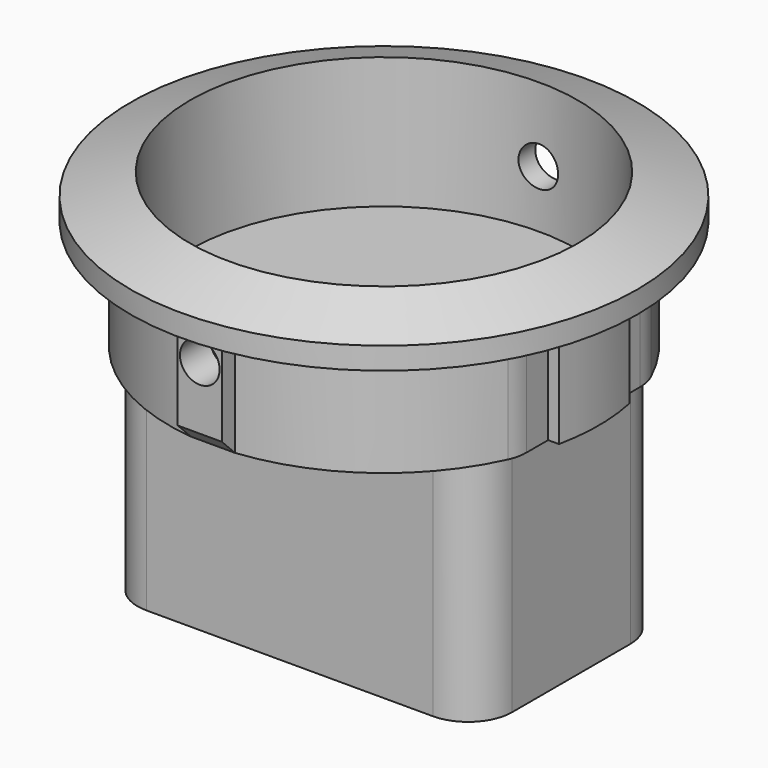
from build123d import *

# Parameters (mm, degrees)
F0_R      = 11.5
F1_DEPTH  = 2
F3_DEPTH  = 5
F5_DEPTH  = 10.5
F6_W      = 0.8
F6_H      = 5
F7_DEPTH  = 5
F8_R      = 8.8
F9_DEPTH  = 6
F11_R     = 2
F12_SIZE  = 0.75
F13_R     = 0.9
F14_DEPTH = 21.9495823706


# Not quite as in the source:
# - a fillet or chamfer that OpenCascade refuses, or shapes differently, is made with other operations: its cross-section is extruded or revolved along the edge and cut away or added


with BuildPart() as f1:
    # F0 (on Top) → F1 (new body)
    with BuildSketch(Plane.XY):
        Circle(F0_R)
    extrude(amount=F1_DEPTH)

    # F2 (on face) → F3 (join)
    with BuildSketch(Plane(origin=(0, 0, 0), x_dir=(1, 0, 0), z_dir=(0, 0, -1))):
        with BuildLine():
            Line((-9.05, -2), (-9.05, -3.6276714294))
            ThreePointArc((-9.05, -3.6276714294), (0, -9.75), (9.05, -3.6276714294))
            Line((9.05, -3.6276714294), (9.05, -2))
            Line((9.05, -2), (9.05, 2))
            Line((9.05, 2), (9.05, 3.6276714294))
            ThreePointArc((9.05, 3.6276714294), (5.8706571109, 7.7844643416), (1, 9.6985823706))
            Line((1, 9.6985823706), (1, 10.4485823706))
            Line((1, 10.4485823706), (-1, 10.4485823706))
            Line((-1, 10.4485823706), (-1, 9.6985823706))
            ThreePointArc((-1, 9.6985823706), (-5.8706571109, 7.7844643416), (-9.05, 3.6276714294))
            Line((-9.05, 3.6276714294), (-9.05, 2))
            Line((-9.05, 2), (-9.05, -2))
        make_face()
        with BuildLine():
            Line((-9.542667342, -2), (-9.05, -2))
            Line((-9.05, -2), (-9.05, 2))
            Line((-9.05, 2), (-9.542667342, 2))
            ThreePointArc((-9.542667342, 2), (-9.75, 0), (-9.542667342, -2))
        make_face()
        with BuildLine():
            Line((9.05, 2), (9.05, -2))
            Line((9.05, -2), (9.542667342, -2))
            ThreePointArc((9.542667342, -2), (9.75, 0), (9.542667342, 2))
            Line((9.542667342, 2), (9.05, 2))
        make_face()
    extrude(amount=F3_DEPTH)

    # F4 (on face) → F5 (join)
    with BuildSketch(Plane(origin=(0, 0, -5), x_dir=(1, 0, 0), z_dir=(0, 0, -1))):
        with BuildLine():
            Line((6.5, 5.35), (-6.5, 5.35))
            ThreePointArc((-6.5, 5.35), (-7.9142135624, 4.7642135624), (-8.5, 3.35))
            Line((-8.5, 3.35), (-8.5, -3.35))
            ThreePointArc((-8.5, -3.35), (-7.9142135624, -4.7642135624), (-6.5, -5.35))
            Line((-6.5, -5.35), (6.5, -5.35))
            ThreePointArc((6.5, -5.35), (7.9142135624, -4.7642135624), (8.5, -3.35))
            Line((8.5, -3.35), (8.5, 3.35))
            ThreePointArc((8.5, 3.35), (7.9142135624, 4.7642135624), (6.5, 5.35))
        make_face()
    extrude(amount=F5_DEPTH)

    # F6 (on face) → F7 (cut)
    with BuildSketch(Plane(origin=(0, 0, -15.5), x_dir=(1, 0, 0), z_dir=(0, 0, -1))):
        Rectangle(F6_W, F6_H)
        with Locations((-7.1, 0)):
            Rectangle(F6_W, F6_H)
        with Locations((7.1, 0)):
            Rectangle(F6_W, F6_H)
    extrude(amount=-F7_DEPTH, mode=Mode.SUBTRACT)

    # F8 (on face) → F9 (cut)
    with BuildSketch(Plane.XY.offset(2)):
        Circle(F8_R)
    extrude(amount=-F9_DEPTH, mode=Mode.SUBTRACT)

    # F10: chamfer of 2.8 x 1 on 1 edges, made by hand

    # F10_s1 → F10_t2 (revolve, cut)
    with BuildSketch(Plane.XZ):
        Polygon((11.5, 1), (8.7, 2), (11.5, 2), align=None)
    revolve(axis=Axis((0, 0, 2), (0, 0, 1)), mode=Mode.SUBTRACT)

    # F11
    f11_edges = [f1.edges().sort_by_distance(p)[0] for p in [
        (-9.05, 3.627671, -2.5),
        (-9.05, -3.627671, -2.5),
        (9.05, -3.627671, -2.5),
        (9.05, 3.627671, -2.5),
    ]]
    fillet(f11_edges, radius=F11_R)

    # F12
    f12_edges = [f1.edges().sort_by_distance(p)[0] for p in [
        (0, -10.448582, -5),
    ]]
    chamfer(f12_edges, length=F12_SIZE)

    # F13 (on face) → F14 (cut, through all)
    with BuildSketch(Plane.XZ.offset(10.4485823706)):
        with Locations((0, -1.4)):
            Circle(F13_R)
    extrude(amount=-F14_DEPTH, mode=Mode.SUBTRACT)


solid = f1.part
